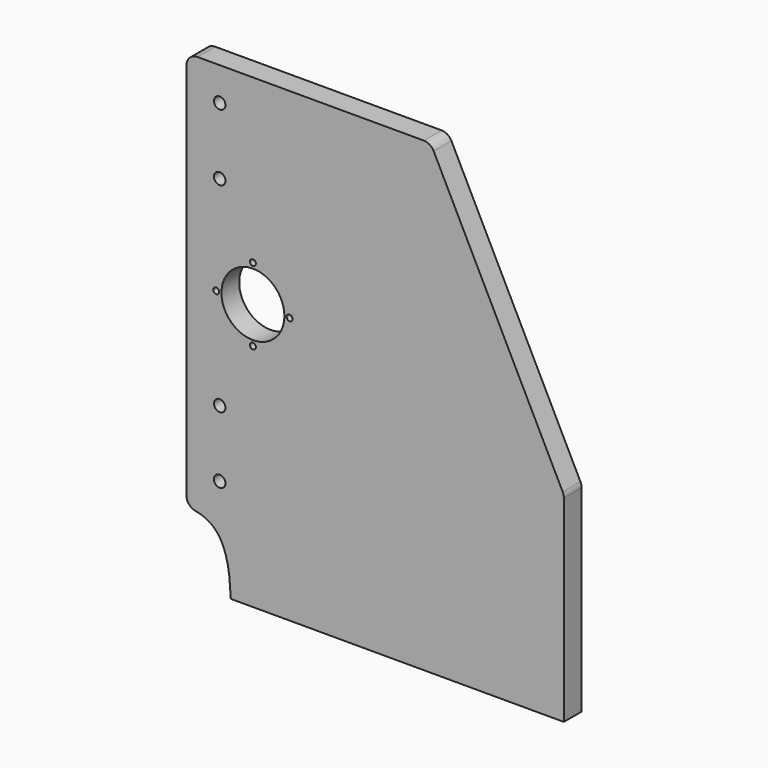
from build123d import *

# Parameters (mm, degrees)
F0_R     = 3.302
F0_R_2   = 1.7
F0_R_3   = 18
F1_DEPTH = 12.7
F2_DEPTH = 25.4
F4_R     = 6.35
F3_R     = 1.7
F5_DEPTH = 12.7
F6_R     = 2.7051
F7_DEPTH = 25.4


# Not quite as in the source:
# - a feature names something its author has since deleted; it is built from what else it names


with BuildPart() as f1:
    # F0 (on Front) → F1 (new body)
    with BuildSketch(Plane.XZ):
        with BuildLine():
            Line((108.4265169831, 0.0004552842), (32.2265169831, 152.4004552842))
            Line((32.2265169831, 152.4004552842), (-107.4734830169, 152.4004552842))
            Line((-107.4734830169, 152.4004552842), (-107.4734830169, -76.1995447158))
            add(Edge.make_bspline(
                [(-82.0734830169, -114.2995447158), (-82.8863746009, -95.7832909802), (-85.4194185281, -76.1871889735), (-107.4734830169, -76.1995447158)],
                knots=[0, 0, 0, 0, 45.7905011984, 45.7905011984, 45.7905011984, 45.7905011984], degree=3))
            Line((-82.0734830169, -114.2995447158), (108.4265169831, -114.2995447158))
            Line((108.4265169831, -114.2995447158), (108.4265169831, 0.0004552842))
        make_face()
        with Locations((-88.4234830169, -57.1371889735)):
            Circle(F0_R, mode=Mode.SUBTRACT)
        with Locations((-88.4234830169, -19.0371889735)):
            Circle(F0_R, mode=Mode.SUBTRACT)
        with Locations((-92.9944827628, 14.5430932346)):
            Circle(F0_R_2, mode=Mode.SUBTRACT)
        with Locations((-69.4244827628, 17.1130932346)):
            Circle(F0_R_2, mode=Mode.SUBTRACT)
        with Locations((-45.8544827628, 14.5430932346)):
            Circle(F0_R_2, mode=Mode.SUBTRACT)
        with Locations((-90.4244827628, 38.1130932346)):
            Circle(F0_R_2, mode=Mode.SUBTRACT)
        with Locations((-69.4244827628, 38.1130932346)):
            Circle(F0_R_3, mode=Mode.SUBTRACT)
        with Locations((-92.9944827628, 61.6830932346)):
            Circle(F0_R_2, mode=Mode.SUBTRACT)
        with Locations((-69.4244827628, 59.1130932346)):
            Circle(F0_R_2, mode=Mode.SUBTRACT)
        with Locations((-48.4244827628, 38.1130932346)):
            Circle(F0_R_2, mode=Mode.SUBTRACT)
        with Locations((-45.8544827628, 61.6830932346)):
            Circle(F0_R_2, mode=Mode.SUBTRACT)
        with Locations((-88.4234830169, 95.2504552842)):
            Circle(F0_R, mode=Mode.SUBTRACT)
        with Locations((-88.4234830169, 133.3504552842)):
            Circle(F0_R, mode=Mode.SUBTRACT)
        with Locations((-92.9944827628, 14.5430932346)):
            Circle(F0_R_2)
        with Locations((-45.8544827628, 61.6830932346)):
            Circle(F0_R_2)
    extrude(amount=F1_DEPTH)

    # F0 (on Front) → F2 (cut)
    with BuildSketch(Plane.XZ):
        with BuildLine():
            add(Edge.make_bspline(
                [(-82.0734830169, -114.2995447158), (-82.8863746009, -95.7832909802), (-85.4194185281, -76.1871889735), (-107.4734830169, -76.1995447158)],
                knots=[0, 0, 0, 0, 45.7905011984, 45.7905011984, 45.7905011984, 45.7905011984], degree=3))
            Line((-107.4734830169, -76.1995447158), (-107.4734830169, -114.2995447158))
            Line((-107.4734830169, -114.2995447158), (-82.0734830169, -114.2995447158))
        make_face()
        with BuildLine():
            Line((108.4265169831, 0.0004552842), (32.2265169831, 152.4004552842))
            Line((32.2265169831, 152.4004552842), (-107.4734830169, 152.4004552842))
            Line((-107.4734830169, 152.4004552842), (-107.4734830169, -76.1995447158))
            add(Edge.make_bspline(
                [(-82.0734830169, -114.2995447158), (-82.8863746009, -95.7832909802), (-85.4194185281, -76.1871889735), (-107.4734830169, -76.1995447158)],
                knots=[0, 0, 0, 0, 45.7905011984, 45.7905011984, 45.7905011984, 45.7905011984], degree=3))
            Line((-82.0734830169, -114.2995447158), (108.4265169831, -114.2995447158))
            Line((108.4265169831, -114.2995447158), (108.4265169831, 0.0004552842))
        make_face()
        with Locations((-88.4234830169, -57.1371889735)):
            Circle(F0_R, mode=Mode.SUBTRACT)
        with Locations((-88.4234830169, -19.0371889735)):
            Circle(F0_R, mode=Mode.SUBTRACT)
        with Locations((-92.9944827628, 14.5430932346)):
            Circle(F0_R_2, mode=Mode.SUBTRACT)
        with Locations((-69.4244827628, 17.1130932346)):
            Circle(F0_R_2, mode=Mode.SUBTRACT)
        with Locations((-45.8544827628, 14.5430932346)):
            Circle(F0_R_2, mode=Mode.SUBTRACT)
        with Locations((-90.4244827628, 38.1130932346)):
            Circle(F0_R_2, mode=Mode.SUBTRACT)
        with Locations((-69.4244827628, 38.1130932346)):
            Circle(F0_R_3, mode=Mode.SUBTRACT)
        with Locations((-92.9944827628, 61.6830932346)):
            Circle(F0_R_2, mode=Mode.SUBTRACT)
        with Locations((-69.4244827628, 59.1130932346)):
            Circle(F0_R_2, mode=Mode.SUBTRACT)
        with Locations((-48.4244827628, 38.1130932346)):
            Circle(F0_R_2, mode=Mode.SUBTRACT)
        with Locations((-45.8544827628, 61.6830932346)):
            Circle(F0_R_2, mode=Mode.SUBTRACT)
        with Locations((-88.4234830169, 95.2504552842)):
            Circle(F0_R, mode=Mode.SUBTRACT)
        with Locations((-88.4234830169, 133.3504552842)):
            Circle(F0_R, mode=Mode.SUBTRACT)
    extrude(amount=-F2_DEPTH, mode=Mode.SUBTRACT)

    # F4
    f4_edges = [f1.edges().sort_by_distance(p)[0] for p in [
        (-107.473483, -6.35, -76.199545),
        (-107.473483, -6.35, 152.400455),
        (108.426517, -6.35, 0.000455),
        (32.226517, -6.35, 152.400455),
    ]]
    fillet(f4_edges, radius=F4_R)

    # F3 (on face) → F5 (join)
    with BuildSketch(Plane.XZ.offset(12.7)):
        with Locations((-45.8544827628, 14.5430932346)):
            Circle(F3_R)
        with Locations((-92.9944827628, 61.6830932346)):
            Circle(F3_R)
    extrude(amount=-F5_DEPTH)

    # F6 (on face) → F7 (cut)
    with BuildSketch(Plane(origin=(0, 0, -114.2995447158), x_dir=(1, 0, 0), z_dir=(0, 0, -1))):
        with Locations((-69.3734830169, 6.35)):
            Circle(F6_R)
        with Locations((-28.0984830169, 6.35)):
            Circle(F6_R)
        with Locations((13.1765169831, 6.35)):
            Circle(F6_R)
        with Locations((54.4515169831, 6.35)):
            Circle(F6_R)
        with Locations((95.7265169831, 6.35)):
            Circle(F6_R)
    extrude(amount=-F7_DEPTH, mode=Mode.SUBTRACT)


solid = f1.part
